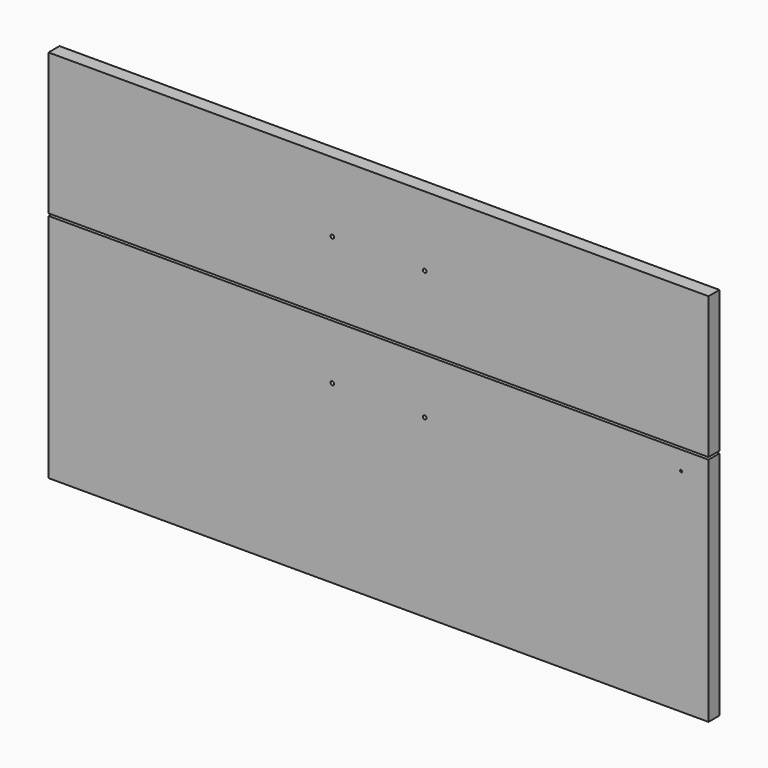
from build123d import *

# Parameters (mm, degrees)
F0_W     = 914.4
F0_H     = 519.176
F1_DEPTH = 19.05
F3_D     = 5.0038
F3_DEPTH = 25.4
F3_TIP   = 1.5032931827
F5_D     = 3.175
F5_DEPTH = 14.224
F5_TIP   = 0.9538662327
F6_W     = 914.4
F6_H     = 3.175
F7_DEPTH = 25.4


with BuildPart() as f1:
    # F0 (on Front) → F1 (new body)
    with BuildSketch(Plane.XZ):
        Rectangle(F0_W, F0_H)
    extrude(amount=F1_DEPTH)

    # F3
    with Locations(Plane.XZ.offset(19.05)):
        with Locations((-64.008, 162.814), (64.008, 162.814), (-64.008, -16.002), (64.008, -16.002)):
            Hole(F3_D / 2, depth=F3_DEPTH)
            with Locations((0, 0, -(F3_DEPTH + F3_TIP / 2))):  # 118° drill point
                Cone(0, F3_D / 2, F3_TIP, mode=Mode.SUBTRACT)

    # F5
    with Locations(Plane.XZ.offset(19.05)):
        with Locations((419.1, 34.036)):
            Hole(F5_D / 2, depth=F5_DEPTH)
            with Locations((0, 0, -(F5_DEPTH + F5_TIP / 2))):  # 118° drill point
                Cone(0, F5_D / 2, F5_TIP, mode=Mode.SUBTRACT)

    # F6 (on face) → F7 (cut)
    with BuildSketch(Plane.XZ.offset(19.05)):
        with Locations((0, 61.7855)):
            Rectangle(F6_W, F6_H)
    extrude(amount=-F7_DEPTH, mode=Mode.SUBTRACT)


solid = f1.part
